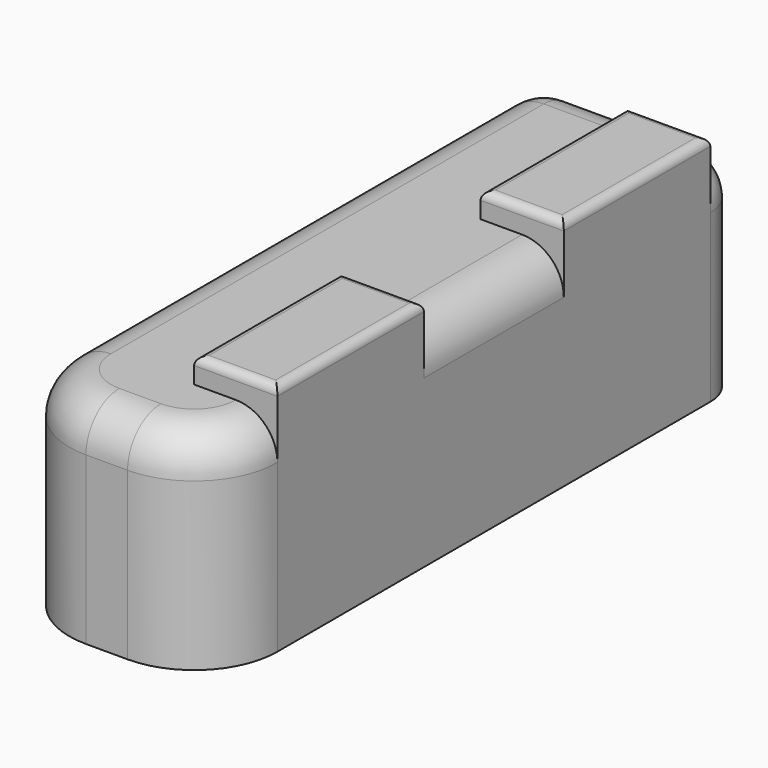
from build123d import *

# Parameters (mm, degrees)
F1_DEPTH = 25
F2_W     = 10
F2_H     = 22
F3_DEPTH = 3
F4_R     = 4.99999
F5_R     = 1


# Not quite as in the source:
# - a fillet or chamfer is up to 0.001 mm smaller than in the source, because OpenCascade refuses the exact size


with BuildPart() as f1:
    # F0 (on Top) → F1 (new body)
    with BuildSketch(Plane.XY):
        with BuildLine():
            Line((0, 54.0433624494), (0, 53.3714158042))
            Line((0, 53.3714158042), (25, 53.3714158042))
            Line((25, 53.3714158042), (25, 54.0433624494))
            ThreePointArc((25, 54.0433624494), (23.5355339059, 57.5788963554), (20, 59.0433624494))
            Line((20, 59.0433624494), (5, 59.0433624494))
            ThreePointArc((5, 59.0433624494), (1.4644660941, 57.5788963554), (0, 54.0433624494))
        make_face()
        with BuildLine():
            Line((25, 53.3714158042), (0, 53.3714158042))
            Line((0, 53.3714158042), (0, -10.9566375506))
            ThreePointArc((0, -10.9566375506), (2.9289321881, -18.0277053624), (10, -20.9566375506))
            Line((10, -20.9566375506), (15, -20.9566375506))
            ThreePointArc((15, -20.9566375506), (22.0710678119, -18.0277053624), (25, -10.9566375506))
            Line((25, -10.9566375506), (25, 53.3714158042))
        make_face()
    extrude(amount=F1_DEPTH)

    # F2 (on face) → F3 (join)
    with BuildSketch(Plane.XY.offset(25)):
        with Locations((20, 0.0433624494)):
            Rectangle(F2_W, F2_H)
        with Locations((20, 43.0433624494)):
            Rectangle(F2_W, F2_H)
    extrude(amount=F3_DEPTH)

    # F4 (radius 5 in the source; OpenCascade refuses exactly that, so slightly less here)
    f4_edges = [f1.edges().sort_by_distance(p)[0] for p in [
        (25, 21.543362, 25),
        (0, 21.543362, 25),
    ]]
    fillet(f4_edges, radius=F4_R)

    # F5
    f5_edges = [f1.edges().sort_by_distance(p)[0] for p in [
        (15, 0.043362, 28),
        (20, -10.956638, 28),
        (25, 0.043362, 28),
        (20, 11.043362, 28),
        (25, 43.043362, 28),
        (20, 54.043362, 28),
        (15, 43.043362, 28),
        (20, 32.043362, 28),
    ]]
    fillet(f5_edges, radius=F5_R)


solid = f1.part
